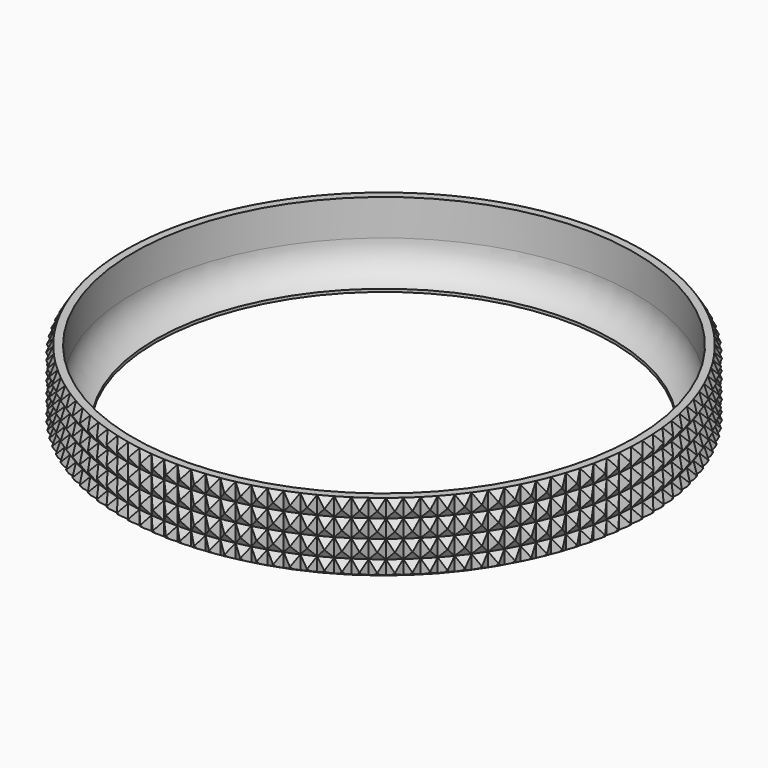
from build123d import *

# Parameters (mm, degrees)
F3_DEPTH        = 7.621
F3_COPIES_COUNT = 120


# Not quite as in the source:
# - a pattern or mirror of a feature is missing from the dataset's text; its kind, count and spacing are read off the source's solid


with BuildPart() as f1:
    # F0 (on Front) → F1 (revolve)
    with BuildSketch(Plane.XZ):
        with BuildLine():
            Line((24.1513906842, 0), (27.2795, 0))
            Line((27.2795, 0), (27.2795, 1.905))
            Line((27.2795, 1.905), (27.2795, 3.81))
            Line((27.2795, 3.81), (27.2795, 5.715))
            Line((27.2795, 5.715), (27.2795, 7.62))
            Line((27.2795, 7.62), (26.4795, 7.62))
            Line((26.4795, 7.62), (26.4795, 3.81))
            ThreePointArc((26.4795, 3.81), (25.8445672046, 1.7040445763), (24.1513906842, 0.3))
            Line((24.1513906842, 0.3), (24.1513906842, 0))
        make_face()
        Polygon((27.2795, 1.905), (27.2795, 0), (27.8795, 0.9525), align=None)
        Polygon((27.2795, 3.81), (27.2795, 1.905), (27.8795, 2.8575), align=None)
        Polygon((27.2795, 5.715), (27.2795, 3.81), (27.8795, 4.7625), align=None)
        Polygon((27.2795, 7.62), (27.2795, 5.715), (27.8795, 6.6675), align=None)
    revolve(axis=Axis((0, 0, 1.8219693994), (0, 0, 1)))

    # F2 (on Top) → F3 (cut, through all)
    with BuildSketch(Plane.XY):
        Polygon((0.7300504004, -27.8795), (0, -27.2795), (-0.7300504004, -27.8795), align=None)
    f3 = extrude(amount=F3_DEPTH, mode=Mode.SUBTRACT)

    # F3_copies: F3 ×120 about axis
    f3_copies_axis = Axis((0, 0, 0), (0, 0, 1))
    for i in range(1, F3_COPIES_COUNT):
        add(f3.rotate(f3_copies_axis, i * 360 / F3_COPIES_COUNT), mode=Mode.SUBTRACT)

    # F4 (on Front) → F5 (revolve, cut)
    with BuildSketch(Plane.XZ):
        Polygon((27.7204448819, 0.7), (26.5080093166, 0), (27.7204448819, 0), align=None)
    revolve(axis=Axis((0, 0, 1.8219693994), (0, 0, 1)), mode=Mode.SUBTRACT)


solid = f1.part
